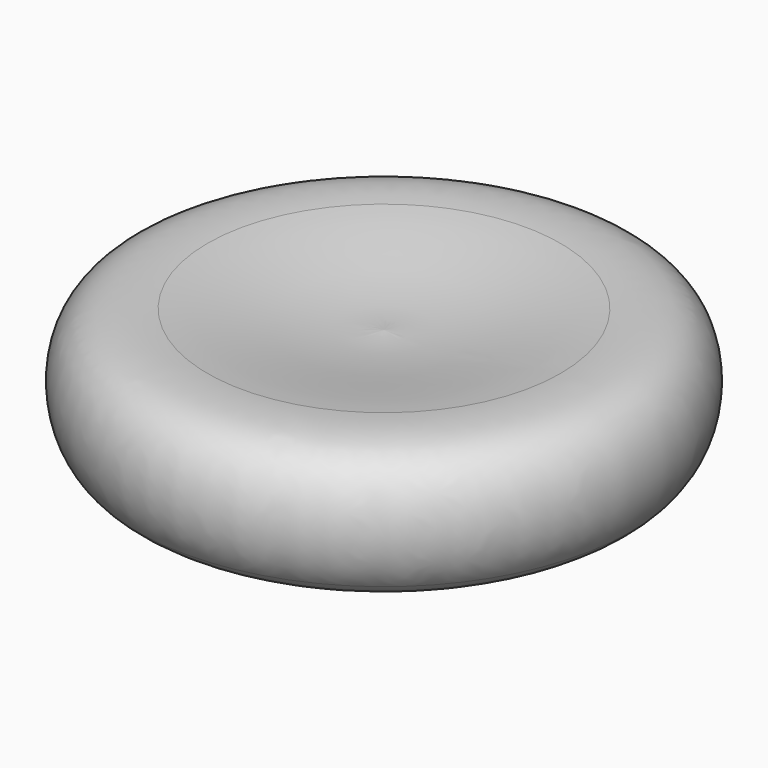
from build123d import *


with BuildPart() as f1:
    # F0 (on Front) → F1 (revolve)
    with BuildSketch(Plane.XZ):
        with BuildLine():
            add(Edge.make_bspline(
                [(8.6320897977, 19.663014639), (6.0541517535, 19.4282337373), (2.717590895, 18.4518785373), (0, 18.7391523166)],
                knots=[0.7524080659, 0.7524080659, 0.7524080659, 0.7524080659, 1, 1, 1, 1], degree=3))
            Line((0, 18.7391523166), (0, 13.2617436071))
            add(Edge.make_bspline(
                [(0, 13.2617436071), (5.787545428, 13.1549302804), (10.2648338323, 11.8778262533), (12.0566570475, 13.9532882355)],
                knots=[0, 0, 0, 0, 0.377777142, 0.377777142, 0.377777142, 0.377777142], degree=3))
            add(Edge.make_bspline(
                [(12.0566570475, 13.9532882355), (13.2364685255, 15.3198593615), (13.2598723957, 19.5671219916), (9.9428268493, 19.7823875725), (8.6320897977, 19.663014639)],
                knots=[0.377777142, 0.377777142, 0.377777142, 0.377777142, 0.6265214402, 0.7524080659, 0.7524080659, 0.7524080659, 0.7524080659], degree=3))
        make_face()
    revolve(axis=Axis((0, 0, -3.2709501684), (0, 0, -1)))


solid = f1.part
